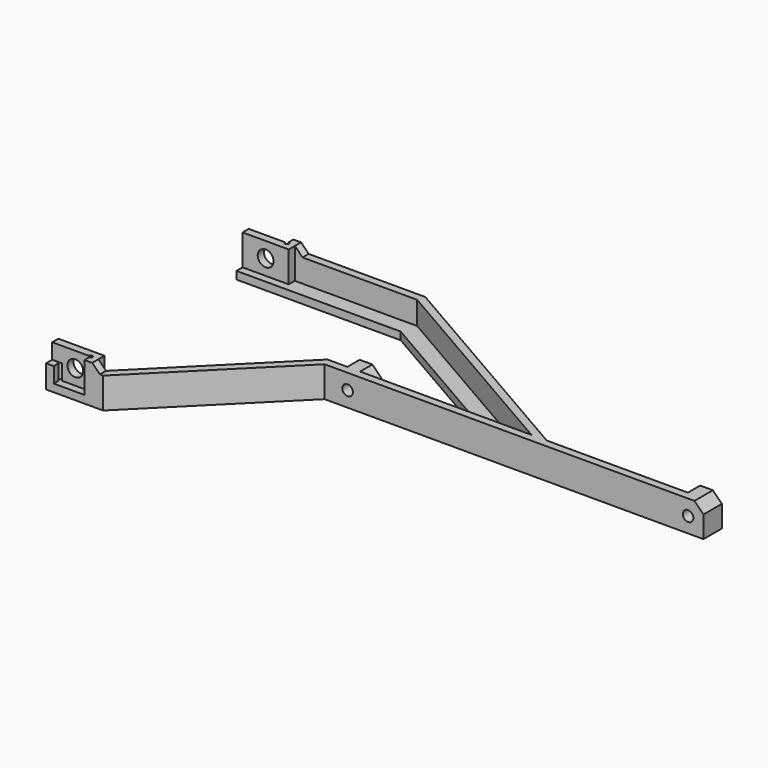
from build123d import *

# Parameters (mm, degrees)
F1_DEPTH  = 1.5875
F3_DEPTH  = 4.7625
F4_W      = 6.35
F4_H      = 6.35
F5_DEPTH  = 3.175
F6_SIZE   = 1.8598642
F7_W      = 42.2204719395
F7_H      = 3.175
F8_DEPTH  = 1.5875
F9_W      = 6.35
F9_H      = 1.5875
F10_DEPTH = 6.35
F11_R     = 1.0922
F11_R_2   = 1.63322
F12_DEPTH = 28.575
F13_SIZE  = 1.58749
F14_R     = 0.396875
F15_DEPTH = 6.35
F16_R     = 1.63322
F17_DEPTH = 1.5875
F18_W     = 138.5852359697
F18_H     = 53.8887336135
F19_DEPTH = 7.9375
F20_W     = 1.5875
F20_H     = 3.175
F21_DEPTH = 1.5875
F22_R     = 0.396875
F23_DEPTH = 3.175


# Not quite as in the source:
# - a fillet or chamfer is up to 0.001 mm smaller than in the source, because OpenCascade refuses the exact size


with BuildPart() as f1:
    # F0 (on Top) → F1 (new body)
    with BuildSketch(Plane.XY):
        Polygon((-87.87765, 25.4), (-127, 25.4), (-127, 20.6375), (-48.7553, 20.6375), (-23.3553, -4.7625), (23.3553, -4.7625), (48.7553, 20.6375), (127, 20.6375), (127, 25.4), (87.87765, 25.4), (46.7826079092, 49.1262336135), (-46.7826079092, 49.1262336135), align=None)
        Polygon((-21.3826079092, 0), (-46.7826079092, 25.4), (-78.35265, 25.4), (-45.5064998802, 44.3637336135), (45.5064998802, 44.3637336135), (78.35265, 25.4), (46.7826079092, 25.4), (21.3826079092, 0), align=None, mode=Mode.SUBTRACT)
    extrude(amount=F1_DEPTH)

    # F2 (on face) → F3 (join)
    with BuildSketch(Plane.XY.offset(1.5875)):
        Polygon((-127, 22.225), (-127, 20.6375), (-48.7553, 20.6375), (-23.3553, -4.7625), (23.3553, -4.7625), (48.7553, 20.6375), (127, 20.6375), (127, 22.225), (93.376911314, 22.225), (87.87765, 25.4), (46.7826079092, 49.1262336135), (-46.7826079092, 49.1262336135), (-87.87765, 25.4), (-93.376911314, 22.225), align=None)
        Polygon((90.201911314, 22.225), (48.0977359697, 22.225), (22.6977359697, -3.175), (21.1102359697, -3.175), (21.1102359697, -1.5875), (-21.1102359697, -1.5875), (-21.1102359697, -3.175), (-22.6977359697, -3.175), (-48.0977359697, 22.225), (-90.201911314, 22.225), (-46.3572385662, 47.5387336135), (-21.1102359697, 47.5387336135), (-21.1102359697, 45.9512336135), (21.1102359697, 45.9512336135), (21.1102359697, 47.5387336135), (46.3572385662, 47.5387336135), align=None, mode=Mode.SUBTRACT)
    extrude(amount=F3_DEPTH)

    # F4 (on face) → F5 (join, through all)
    with BuildSketch(Plane(origin=(0, 22.225, 0), x_dir=(-1, 0, 0), z_dir=(0, 1, 0))):
        with Locations((-53.5178, 3.175)):
            Rectangle(F4_W, F4_H)
        with Locations((-123.825, 3.175)):
            Rectangle(F4_W, F4_H)
        with Locations((123.825, 3.175)):
            Rectangle(F4_W, F4_H)
        with Locations((53.5178, 3.175)):
            Rectangle(F4_W, F4_H)
    extrude(amount=F5_DEPTH)

    # F6
    f6_edges = [f1.edges().sort_by_distance(p)[0] for p in [
        (-127, 23.01875, 6.35),
        (-120.65, 23.8125, 6.35),
        (-56.6928, 23.8125, 6.35),
        (-50.3428, 23.8125, 6.35),
        (50.3428, 23.8125, 6.35),
        (56.6928, 23.8125, 6.35),
        (120.65, 23.8125, 6.35),
        (127, 23.01875, 6.35),
    ]]
    chamfer(f6_edges, length=F6_SIZE)

    # F7 (on face) → F8 (join)
    with BuildSketch(Plane.XY.offset(6.35)):
        with Locations((0, -3.175)):
            Rectangle(F7_W, F7_H)
        with Locations((0, 47.5387336135)):
            Rectangle(F7_W, F7_H)
    extrude(amount=F8_DEPTH)

    # F9 (on face) → F10 (cut, through all)
    with BuildSketch(Plane.XY.offset(7.9375)):
        with Locations((16.3477359697, -3.96875)):
            Rectangle(F9_W, F9_H)
        with Locations((16.3477359697, 48.3324836135)):
            Rectangle(F9_W, F9_H)
    extrude(amount=-F10_DEPTH, mode=Mode.SUBTRACT)

    # F11 (on face) → F12 (cut, through all)
    with BuildSketch(Plane.XZ.offset(3.175)):
        with Locations((53.5178, 3.175)):
            Circle(F11_R)
        with Locations((123.825, 3.175)):
            Circle(F11_R)
        with Locations((-123.825, 3.175)):
            Circle(F11_R)
        with Locations((-53.5178, 3.175)):
            Circle(F11_R)
        with Locations((16.3477359697, 4.7625)):
            Circle(F11_R_2)
    extrude(amount=-F12_DEPTH, mode=Mode.SUBTRACT)

    # F13 (size 1.5875 in the source; OpenCascade refuses exactly that, so slightly less here)
    f13_edges = [f1.edges().sort_by_distance(p)[0] for p in [
        (-21.110236, -3.96875, 6.35),
        (21.110236, -3.96875, 6.35),
        (-21.110236, 48.332484, 6.35),
        (21.110236, 48.332484, 6.35),
    ]]
    chamfer(f13_edges, length=F13_SIZE)

    # F14 (on face) → F15 (cut, through all)
    with BuildSketch(Plane.XY.offset(7.9375)):
        with Locations((19.5227359697, -3.175)):
            Circle(F14_R)
        with Locations((19.5227359697, 47.5387336135)):
            Circle(F14_R)
    extrude(amount=-F15_DEPTH, mode=Mode.SUBTRACT)

    # F16 (on face) → F17 (cut, through all)
    with BuildSketch(Plane(origin=(0, 47.5387336135, 0), x_dir=(-1, 0, 0), z_dir=(0, 1, 0))):
        with Locations((-16.3477359697, 4.7625)):
            Circle(F16_R)
    extrude(amount=-F17_DEPTH, mode=Mode.SUBTRACT)

    # F18 (on face) → F19 (cut, through all)
    with BuildSketch(Plane.XY.offset(7.9375)):
        with Locations((-57.7073820151, 22.1818668067)):
            Rectangle(F18_W, F18_H)
    extrude(amount=-F19_DEPTH, mode=Mode.SUBTRACT)

    # F20 (on face) → F21 (cut, through all)
    with BuildSketch(Plane.YZ.offset(13.1727359697)):
        with Locations((48.3324836135, 6.35)):
            Rectangle(F20_W, F20_H)
        with Locations((-3.96875, 6.35)):
            Rectangle(F20_W, F20_H)
    extrude(amount=-F21_DEPTH, mode=Mode.SUBTRACT)

    # F22 (on face) → F23 (cut, through all)
    with BuildSketch(Plane.XY.offset(4.7625)):
        with Locations((13.1727359697, -3.175)):
            Circle(F22_R)
        with Locations((13.1727359697, 47.5387336135)):
            Circle(F22_R)
    extrude(amount=-F23_DEPTH, mode=Mode.SUBTRACT)


solid = f1.part
